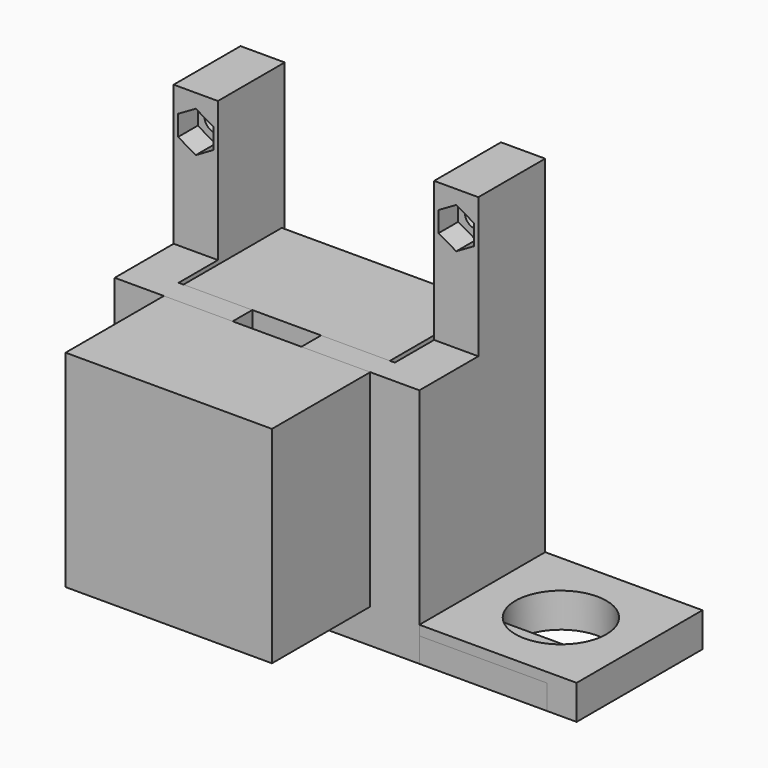
from build123d import *

# Parameters (mm, degrees)
F1_R      = 2.25
F2_DEPTH  = 12
F4_DEPTH  = 5
F5_W      = 44
F5_H      = 10
F5_H_2    = 5
F6_DEPTH  = 7
F7_DEPTH  = 42
F8_R      = 1.7
F8_R_2    = 13
F9_DEPTH  = 5
F11_REACH = 63.8670687473
F12_R     = 1.7
F13_DEPTH = 25
F14_W     = 42
F14_H     = 42
F14_R     = 1.7
F14_R_2   = 13
F15_DEPTH = 25
F16_W     = 32
F16_H     = 32
F16_R     = 9.25
F17_DEPTH = 7
F18_W     = 26
F18_H     = 12
F19_DEPTH = 5
F20_D     = 3.3


with BuildPart() as f2:
    # F1 (on Front) → F2 (new body)
    with BuildSketch(Plane.XZ):
        Polygon((-27, 56.5), (-36, 56.5), (-36, -21), (26, -21), (26, 56.5), (17, 56.5), (17, -14), (-27, -14), align=None)
        with Locations((-31.5, 49.5)):
            Circle(F1_R, mode=Mode.SUBTRACT)
        with Locations((21.5, 49.5)):
            Circle(F1_R, mode=Mode.SUBTRACT)
    extrude(amount=-F2_DEPTH)

    # F3 (on face) → F4 (join)
    with BuildSketch(Plane.XZ):
        Polygon((-27, -14), (-27, 56.5), (-36, 56.5), (-36, -21), (26, -21), (26, 56.5), (17, 56.5), (17, -14), align=None)
        Polygon((-31.5, 53.6569219382), (-27.9, 51.5784609691), (-27.9, 47.4215390309), (-31.5, 45.3430780618), (-35.1, 47.4215390309), (-35.1, 51.5784609691), align=None, mode=Mode.SUBTRACT)
        Polygon((21.5, 53.6569219382), (25.1, 51.5784609691), (25.1, 47.4215390309), (21.5, 45.3430780618), (17.9, 47.4215390309), (17.9, 51.5784609691), align=None, mode=Mode.SUBTRACT)
    extrude(amount=F4_DEPTH)

    # F5 (on face) → F6 (join, through all)
    with BuildSketch(Plane.XY.offset(-14)):
        with Locations((-5, -10)):
            Rectangle(F5_W, F5_H)
        with Locations((-5, -17.5)):
            Rectangle(F5_W, F5_H_2)
        Polygon((-27, -15), (-27, -5), (-36, -5), (-36, -20), (-27, -20), align=None)
        Polygon((26, -5), (17, -5), (17, -15), (17, -20), (26, -20), align=None)
    extrude(amount=-F6_DEPTH)

    # F5 (on face) → F7 (join)
    with BuildSketch(Plane.XY.offset(-14)):
        with Locations((-5, -17.5)):
            Rectangle(F5_W, F5_H_2)
        Polygon((-27, -15), (-27, -5), (-36, -5), (-36, -20), (-27, -20), align=None)
        Polygon((26, -5), (17, -5), (17, -15), (17, -20), (26, -20), align=None)
    extrude(amount=F7_DEPTH)

    # F8 (on face) → F9 (cut, through all)
    with BuildSketch(Plane.XZ.offset(20)):
        with Locations((-20.5, 22.5)):
            Circle(F8_R)
        with Locations((-5, 7)):
            Circle(F8_R_2)
        with Locations((-20.5, -8.5)):
            Circle(F8_R)
        with Locations((10.5, -8.5)):
            Circle(F8_R)
        with Locations((10.5, 22.5)):
            Circle(F8_R)
    extrude(amount=-F9_DEPTH, mode=Mode.SUBTRACT)

    f11_end = f2.faces().sort_by_distance((-18, -17.5, 7))[0]
    # F10 (on face) → F11 (cut, up to a face of the model that its end follows)
    with BuildSketch(Plane.XY.offset(28)):
        Polygon((2, -15), (-5, -15), (-12, -15), (-12, -20), (2, -20), align=None)
    f11_long = extrude(amount=-F11_REACH, mode=Mode.PRIVATE)
    add(split(f11_long, bisect_by=f11_end, keep=Keep.ALL, mode=Mode.PRIVATE).solids().sort_by_distance((-5, -17.5, 28))[0], mode=Mode.SUBTRACT)


with BuildPart() as f13:
    # F12 (on face) → F13 (new body)
    with BuildSketch(Plane(origin=(0, -15, 0), x_dir=(-1, 0, 0), z_dir=(0, 1, 0))):
        with BuildLine():
            Line((-16, -14), (26, -14))
            Line((26, -14), (26, 28))
            Line((26, 28), (12, 28))
            Line((12, 28), (12, 17.9544511501))
            ThreePointArc((12, 17.9544511501), (5, -6), (-2, 17.9544511501))
            Line((-2, 17.9544511501), (-2, 28))
            Line((-2, 28), (-16, 28))
            Line((-16, 28), (-16, -14))
        make_face()
        with Locations((-10.5, -8.5)):
            Circle(F12_R, mode=Mode.SUBTRACT)
        with Locations((20.5, -8.5)):
            Circle(F12_R, mode=Mode.SUBTRACT)
        with Locations((-10.5, 22.5)):
            Circle(F12_R, mode=Mode.SUBTRACT)
        with Locations((20.5, 22.5)):
            Circle(F12_R, mode=Mode.SUBTRACT)
        with BuildLine():
            Line((12, 17.9544511501), (12, 28))
            Line((12, 28), (-2, 28))
            Line((-2, 28), (-2, 17.9544511501))
            ThreePointArc((-2, 17.9544511501), (5, -6), (12, 17.9544511501))
        make_face()
        with Locations((-10.5, 22.5)):
            Circle(F12_R)
        with Locations((20.5, 22.5)):
            Circle(F12_R)
        with Locations((-10.5, -8.5)):
            Circle(F12_R)
        with Locations((20.5, -8.5)):
            Circle(F12_R)
    extrude(amount=F13_DEPTH)


with BuildPart() as f15:
    # F14 (on face) → F15 (new body)
    with BuildSketch(Plane.XZ.offset(20)):
        with Locations((-5, 7)):
            Rectangle(F14_W, F14_H)
        with Locations((-20.5, -8.5)):
            Circle(F14_R, mode=Mode.SUBTRACT)
        with Locations((10.5, -8.5)):
            Circle(F14_R, mode=Mode.SUBTRACT)
        with Locations((-20.5, 22.5)):
            Circle(F14_R, mode=Mode.SUBTRACT)
        with Locations((-5, 7)):
            Circle(F14_R_2, mode=Mode.SUBTRACT)
        with Locations((10.5, 22.5)):
            Circle(F14_R, mode=Mode.SUBTRACT)
    extrude(amount=F15_DEPTH)

    # F8 (on face) → F15, piece 2 (join)
    with BuildSketch(Plane.XZ.offset(20)):
        with Locations((-20.5, 22.5)):
            Circle(F8_R)
    extrude(amount=F15_DEPTH)

    # F8 (on face) → F15, piece 3 (join)
    with BuildSketch(Plane.XZ.offset(20)):
        with Locations((-5, 7)):
            Circle(F8_R_2)
    extrude(amount=F15_DEPTH)

    # F8 (on face) → F15, piece 4 (join)
    with BuildSketch(Plane.XZ.offset(20)):
        with Locations((-20.5, -8.5)):
            Circle(F8_R)
    extrude(amount=F15_DEPTH)

    # F8 (on face) → F15, piece 5 (join)
    with BuildSketch(Plane.XZ.offset(20)):
        with Locations((10.5, 22.5)):
            Circle(F8_R)
    extrude(amount=F15_DEPTH)

    # F8 (on face) → F15, piece 6 (join)
    with BuildSketch(Plane.XZ.offset(20)):
        with Locations((10.5, -8.5)):
            Circle(F8_R)
    extrude(amount=F15_DEPTH)


with BuildPart() as f17:
    # F16 (on face) → F17 (new body, through all)
    with BuildSketch(Plane(origin=(0, 0, -21), x_dir=(1, 0, 0), z_dir=(0, 0, -1))):
        with Locations((42, 4)):
            Rectangle(F16_W, F16_H)
        with Locations((42, 4)):
            Circle(F16_R, mode=Mode.SUBTRACT)
    extrude(amount=-F17_DEPTH)


with BuildPart() as f19:
    # F18 (on face) → F19 (new body)
    with BuildSketch(Plane(origin=(0, 0, -21), x_dir=(1, 0, 0), z_dir=(0, 0, -1))):
        with Locations((39, 14)):
            Rectangle(F18_W, F18_H)
    extrude(amount=-F19_DEPTH)

    # F20 (through all)
    with Locations(Plane(origin=(0, 0, -21), x_dir=(1, 0, 0), z_dir=(0, 0, -1))):
        with Locations((30, 14), (48, 14)):
            Hole(F20_D / 2)


solid = Compound([f2.part, f13.part, f15.part, f17.part, f19.part])
